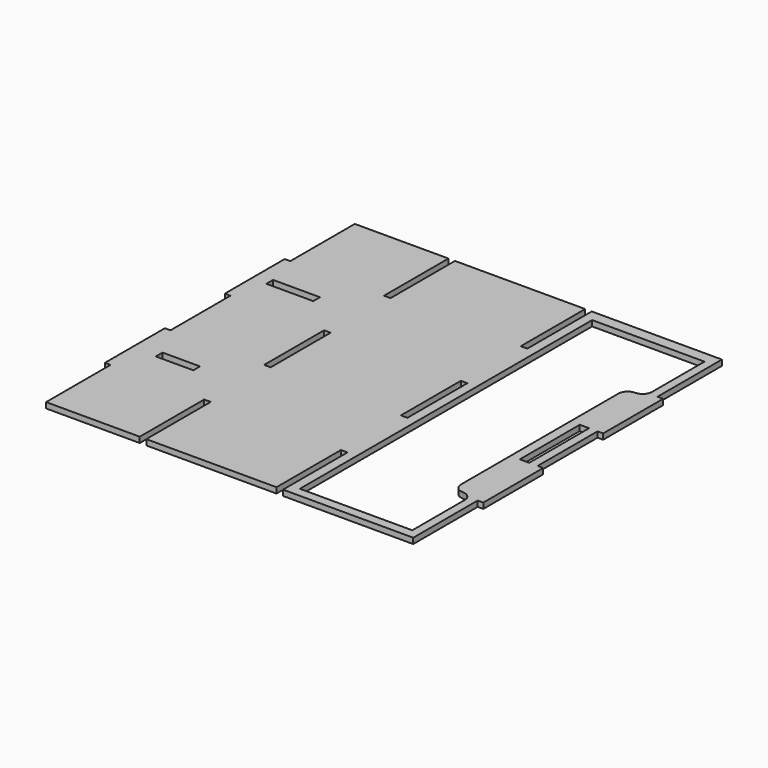
from build123d import *

# Parameters (mm, degrees)
F0_W     = 3.5
F0_H     = 40
F0_W_2   = 5
F1_DEPTH = 3
F2_R     = 4.99999
F3_R     = 4.99999


# Not quite as in the source:
# - a fillet or chamfer is up to 0.001 mm smaller than in the source, because OpenCascade refuses the exact size


with BuildPart() as f1:
    # F0 (on Top) → F1 (new body)
    with BuildSketch(Plane.XY):
        Polygon((129.5, -200), (199, -200), (199, -157), (202, -157), (202, -117), (199, -117), (199, -77), (202, -77), (202, -37), (199, -37), (199, 6), (129.5, 6), (129.5, -37), (126, -37), (126, 6), (56.5, 6), (56.5, -37), (53, -37), (53, 6), (3, 6), (3, -37), (0, -37), (0, -77), (3, -77), (3, -117), (0, -117), (0, -157), (3, -157), (3, -200), (53, -200), (53, -157), (56.5, -157), (56.5, -200), (126, -200), (126, -157), (129.5, -157), align=None)
        Polygon((33, -134.75), (33, -137), (33, -139.25), (13, -139.25), (13, -134.75), align=None, mode=Mode.SUBTRACT)
        with Locations((54.75, -97)):
            Rectangle(F0_W, F0_H, mode=Mode.SUBTRACT)
        with Locations((127.75, -97)):
            Rectangle(F0_W, F0_H, mode=Mode.SUBTRACT)
        Polygon((134.5, -195), (134.5, -97), (134.5, 0), (194.5, 0), (194.5, -40), (184.5, -40), (184.5, -155), (194.5, -155), (194.5, -195), align=None, mode=Mode.SUBTRACT)
        with Locations((192, -97)):
            Rectangle(F0_W_2, F0_H, mode=Mode.SUBTRACT)
        Polygon((33, -54.75), (33, -57), (33, -59.25), (8.0116633326, -59.25), (8.0116633326, -54.75), align=None, mode=Mode.SUBTRACT)
    extrude(amount=F1_DEPTH)

    # F2 (radius 5 in the source; OpenCascade refuses exactly that, so slightly less here)
    f2_edges = [f1.edges().sort_by_distance(p)[0] for p in [
        (194.5, -40, 1.5),
        (184.5, -40, 1.5),
    ]]
    fillet(f2_edges, radius=F2_R)

    # F3 (radius 5 in the source; OpenCascade refuses exactly that, so slightly less here)
    f3_edges = [f1.edges().sort_by_distance(p)[0] for p in [
        (194.5, -155, 1.5),
        (184.5, -155, 1.5),
    ]]
    fillet(f3_edges, radius=F3_R)


solid = f1.part
